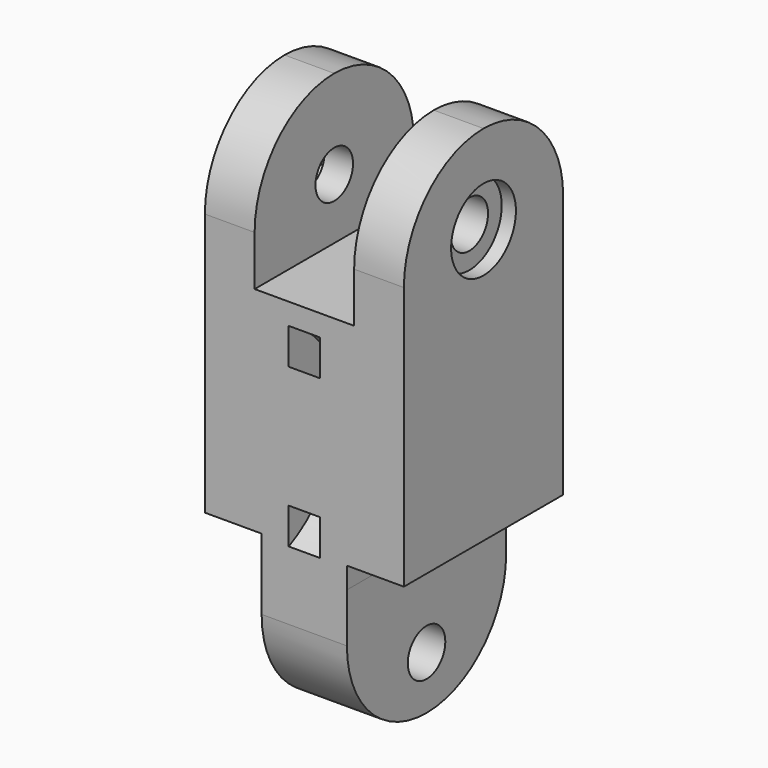
from build123d import *

# Parameters (mm, degrees)
F1_DEPTH  = 7
F2_R      = 1.65
F3_DEPTH  = 25
F4_R      = 1.65
F5_DEPTH  = 25
F6_R      = 6.99999
F7_R      = 2.85
F8_DEPTH  = 1
F10_DEPTH = 1.5
F11_R     = 1.125
F13_R     = 1.125
F16_DEPTH = 25
F19_DEPTH = 1.1


# Not quite as in the source:
# - a fillet or chamfer is up to 0.001 mm smaller than in the source, because OpenCascade refuses the exact size
# - a feature names something its author has since deleted; it is built from what else it names


with BuildPart() as f1:
    # F0 (on Front) → F1 (new body, symmetric)
    with BuildSketch(Plane.XZ):
        Polygon((-39.5, 23.5411238112), (-39.5, 21.5411238112), (-39.5, -1.9508430529), (-35.5, -1.9508430529), (-35.5076822063, -3.4508233807), (-35.5076822063, -6.4508233807), (-29.5076822063, -6.4823476079), (-29.5076822063, -3.4823476079), (-29.5, -1.9823672801), (-25.5, -1.9823672801), (-25.5, 21.5411238112), (-25.5, 23.5411238112), (-29, 23.5411238112), (-29, 21.5334145057), (-29, 13.0334145057), (-36, 13.0334145057), (-36, 21.5411238112), (-36, 23.5411238112), align=None)
        Polygon((-29.5076822063, -6.4823476079), (-35.5076822063, -6.4508233807), (-35.5076822063, -13.9508233807), (-29.5076822063, -13.9508233807), align=None)
    extrude(amount=F1_DEPTH, both=True)

    # F2 (on face) → F3 (cut)
    with BuildSketch(Plane.YZ.offset(-29.5076822063)):
        with Locations((0, -10.2008233807)):
            Circle(F2_R)
    extrude(amount=-F3_DEPTH, mode=Mode.SUBTRACT)

    # F4 (on face) → F5 (cut)
    with BuildSketch(Plane.YZ.offset(-25.5)):
        with Locations((0, 17.2911238112)):
            Circle(F4_R)
    extrude(amount=-F5_DEPTH, mode=Mode.SUBTRACT)

    # F6 (radius 7 in the source; OpenCascade refuses exactly that, so slightly less here)
    f6_edges = [f1.edges().sort_by_distance(p)[0] for p in [
        (-37.75, -7, 23.541124),
        (-37.75, 7, 23.541124),
        (-27.25, 7, 23.541124),
        (-27.25, -7, 23.541124),
        (-32.507682, -7, -13.950823),
        (-32.507682, 7, -13.950823),
    ]]
    fillet(f6_edges, radius=F6_R)

    # F7 (on face) → F8 (cut)
    with BuildSketch(Plane.YZ.offset(-25.5)):
        with Locations((0, 17.2911238112)):
            Circle(F7_R)
    extrude(amount=-F8_DEPTH, mode=Mode.SUBTRACT)

    # F9 (on face) → F10 (cut)
    with BuildSketch(Plane(origin=(-39.5, 0, 0), x_dir=(0, -1, 0), z_dir=(-1, 0, 0))):
        Polygon((-0.0683087897, 14.1156973306), (2.7158456051, 15.6442534237), (2.7841543949, 18.8196799042), (0.0683087897, 20.4665502917), (-2.7158456051, 18.9379941986), (-2.7841543949, 15.7625677181), align=None)
    extrude(amount=-F10_DEPTH, mode=Mode.SUBTRACT)

    # F11 (on face) → F12 (revolve)
    with BuildSketch(Plane.XZ.offset(7)):
        with Locations((-35.5, 7.298982876)):
            Circle(F11_R)
    revolve(axis=Axis((-32.5, -7, 3.0412955625), (0, 0, -1)))

    # F13 (on face) → F14 (revolve)
    with BuildSketch(Plane(origin=(0, 7, 0), x_dir=(-1, 0, 0), z_dir=(0, 1, 0))):
        with Locations((29.6073952019, 7.2832577271)):
            Circle(F13_R)
    revolve(axis=Axis((-32.5, 7, 3.0412955625), (0, 0, -1)))

    # F15 (on face) → F16 (cut)
    with BuildSketch(Plane.XY.offset(13.0334145057)):
        Polygon((-25.5, -7), (-29, -7), (-36, -7), (-39.5, -7), (-39.5, -13.4261082858), (-25.5, -13.4261082858), align=None)
    extrude(amount=-F16_DEPTH, mode=Mode.SUBTRACT)

    # F18 (on offset) → F19 (cut, symmetric)
    with BuildSketch(Plane.YZ.offset(-32.5)):
        with BuildLine():
            ThreePointArc((-7, 9.0029031262), (-4.8, 4.7040660741), (-7, 0.4052290221))
            Line((-7, 0.4052290221), (-7, -2.1252823574))
            ThreePointArc((-7, -2.1252823574), (-2.6, 4.7040660741), (-7, 11.5334145057))
            Line((-7, 11.5334145057), (-7, 9.0029031262))
        make_face()
    extrude(amount=F19_DEPTH, both=True, mode=Mode.SUBTRACT)


solid = f1.part
